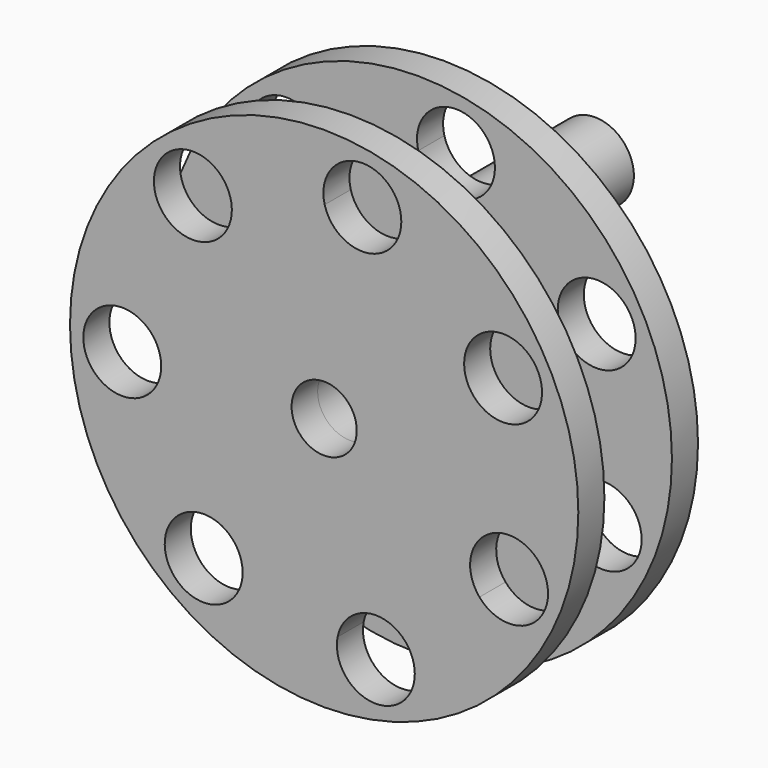
from build123d import *

# Parameters (mm, degrees)
F0_R     = 99.06
F0_R_2   = 12.7
F1_DEPTH = 12.7
F4_R     = 25.7464776051
F4_R_2   = 12.7
F5_DEPTH = 34.29
F6_R     = 15.18285
F7_DEPTH = 58.3057


with BuildPart() as f1:
    # F0 (on Front) → F1 (new body)
    with BuildSketch(Plane.XZ):
        Circle(F0_R)
        with BuildLine():
            ThreePointArc((87.2525606561, -31.7166266483), (77.3287632035, -45.9595652645), (60.5301336512, -41.5835966325))
            Line((60.5301336512, -41.5835966325), (31.6772493906, -66.2543920036))
            ThreePointArc((31.6772493906, -66.2543920036), (34.3806110019, -70.8623094404), (35.3205223857, -76.1213619879))
            ThreePointArc((35.3205223857, -76.1213619879), (18.6961355427, -91.235623652), (5.2285560351, -73.2513125515))
            Line((5.2285560351, -73.2513125515), (-32.0493275742, -66.0752085942))
            ThreePointArc((-32.0493275742, -66.0752085942), (-56.0130922655, -75.3925410567), (-54.0102309185, -49.7592960647))
            Line((-54.0102309185, -49.7592960647), (-71.6421071885, -16.1400454247))
            ThreePointArc((-71.6421071885, -16.1400454247), (-93.8678539395, -3.2136815215), (-72.5782123825, 11.2024852635))
            Line((-72.5782123825, 11.2024852635), (-57.2869188572, 45.9489011465))
            ThreePointArc((-57.2869188572, 45.9489011465), (-61.0382070418, 71.3851457465), (-36.4933195968, 63.7285666992))
            Line((-36.4933195968, 63.7285666992), (0.2064878138, 73.4373879676))
            ThreePointArc((0.2064878138, 73.4373879676), (12.9265601576, 92.3764736183), (30.0672552745, 77.3203859252))
            ThreePointArc((30.0672552745, 77.3203859252), (29.2989487183, 72.551751799), (27.0717871734, 68.2657375846))
            Line((27.0717871734, 68.2657375846), (57.5444049494, 45.6260237994))
            ThreePointArc((57.5444049494, 45.6260237994), (74.5004209745, 50.9859189025), (84.9146368483, 36.5713754587))
            ThreePointArc((84.9146368483, 36.5713754587), (80.649808931, 26.0207485615), (70.2512860382, 21.3974157015))
            Line((70.2512860382, 21.3974157015), (71.5502114662, -16.5426668911))
            ThreePointArc((71.5502114662, -16.5426668911), (82.6203375533, -20.7986045656), (87.2525606561, -31.7166266483))
        make_face(mode=Mode.SUBTRACT)
        with BuildLine():
            Line((31.6772493906, -66.2543920036), (60.5301336512, -41.5835966325))
            ThreePointArc((60.5301336512, -41.5835966325), (58.173043061, -25.6009448486), (71.5502114662, -16.5426668911))
            Line((71.5502114662, -16.5426668911), (70.2512860382, 21.3974157015))
            ThreePointArc((70.2512860382, 21.3974157015), (56.2859237552, 29.519588465), (57.5444049494, 45.6260237994))
            Line((57.5444049494, 45.6260237994), (27.0717871734, 68.2657375846))
            ThreePointArc((27.0717871734, 68.2657375846), (12.0143558381, 62.4112695746), (0.2064878138, 73.4373879676))
            Line((0.2064878138, 73.4373879676), (-36.4933195968, 63.7285666992))
            ThreePointArc((-36.4933195968, 63.7285666992), (-36.1151493645, 61.8034138585), (-35.9883870575, 59.8455687416))
            ThreePointArc((-35.9883870575, 59.8455687416), (-42.8746879342, 47.1299796177), (-57.2869188572, 45.9489011465))
            Line((-57.2869188572, 45.9489011465), (-72.5782123825, 11.2024852635))
            ThreePointArc((-72.5782123825, 11.2024852635), (-65.9783050583, 5.6023667917), (-63.5110441822, -2.6941823316))
            ThreePointArc((-63.5110441822, -2.6941823316), (-65.701874357, -10.5507945139), (-71.6421071885, -16.1400454247))
            Line((-71.6421071885, -16.1400454247), (-54.0102309185, -49.7592960647))
            ThreePointArc((-54.0102309185, -49.7592960647), (-39.1018317425, -50.2131393325), (-31.7755939248, -63.2051591578))
            ThreePointArc((-31.7755939248, -63.2051591578), (-31.8441822607, -64.6466960007), (-32.0493275742, -66.0752085942))
            Line((-32.0493275742, -66.0752085942), (5.2285560351, -73.2513125515))
            ThreePointArc((5.2285560351, -73.2513125515), (16.2546744281, -61.4434445271), (31.6772493906, -66.2543920036))
        make_face()
        Circle(F0_R_2, mode=Mode.SUBTRACT)
    extrude(amount=F1_DEPTH)


with BuildPart() as f2_1:
    # F2: copy of F1
    add(f1.part.moved(Location((0, 30.3657, 0))))


with BuildPart() as f2_1_1:
    # F3: moved
    add(f2_1.part.moved(Location((0, 15.24, 0))))


with BuildPart() as f1_1:
    add(f1.part)

    add(f2_1_1.part)  # F5 merges F2_1
    # F4 (on face) → F5 (join)
    with BuildSketch(Plane(origin=(0, 0, 0), x_dir=(-1, 0, 0), z_dir=(0, 1, 0))):
        Circle(F4_R)
        Circle(F4_R_2, mode=Mode.SUBTRACT)
    extrude(amount=F5_DEPTH)


with BuildPart() as f7:
    # F6 (on face) → F7 (new body)
    with BuildSketch(Plane(origin=(0, 45.6057, 0), x_dir=(-1, 0, 0), z_dir=(0, 1, 0))):
        with Locations((-12.232452631, 44.8086373508)):
            Circle(F6_R)
    extrude(amount=F7_DEPTH)


solid = Compound([f1_1.part, f7.part])
